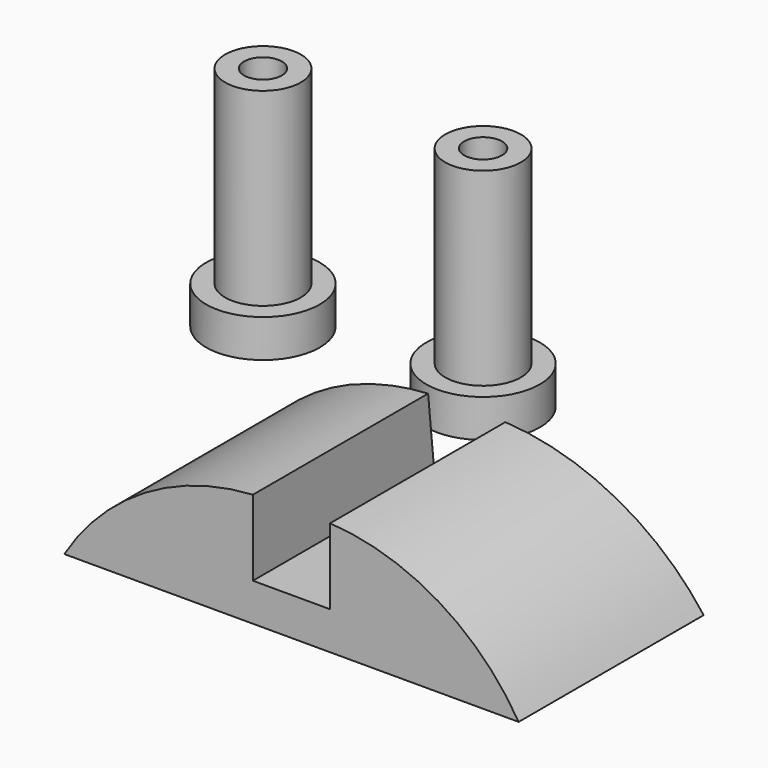
from build123d import *

# Parameters (mm, degrees)
F3_REACH = 81.3802869415
F4_R     = 6.35
F4_R_2   = 3.175
F5_DEPTH = 38.1
F6_R     = 9.525
F7_DEPTH = 6.35


with BuildPart() as f3:
    f3_end = Plane(origin=(0, 38.339396032, 4.1249082693), x_dir=(0, -0.1069719436, 0.9942620395), z_dir=(0, 0.9942620395, 0.1069719436))
    # F1 (on Front) → F3 (new body, up to a plane its end follows)
    with BuildSketch(Plane.XZ):
        with BuildLine():
            Line((0, 6.35), (0, 0))
            Line((0, 0), (38.1, 0))
            ThreePointArc((38.1, 0), (24.6352816359, 13.4206575155), (6.477, 19.05))
            Line((6.477, 19.05), (6.477, 6.35))
            Line((6.477, 6.35), (0, 6.35))
        make_face()
        with BuildLine():
            Line((-38.1, 0), (0, 0))
            Line((0, 0), (0, 6.35))
            Line((0, 6.35), (-6.477, 6.35))
            Line((-6.477, 6.35), (-6.477, 19.05))
            ThreePointArc((-6.477, 19.05), (-24.6352816359, 13.4206575155), (-38.1, 0))
        make_face()
    f3_long = extrude(amount=-F3_REACH, mode=Mode.PRIVATE)
    add(split(f3_long, bisect_by=f3_end, keep=Keep.BOTTOM, mode=Mode.PRIVATE))


with BuildPart() as f5:
    # F4 (on Top) → F5 (new body)
    with BuildSketch(Plane.XY):
        with Locations((-58.1043511629, 66.6491091251)):
            Circle(F4_R)
        with Locations((-58.1043511629, 66.6491091251)):
            Circle(F4_R_2, mode=Mode.SUBTRACT)
    extrude(amount=F5_DEPTH)


with BuildPart() as f5b:
    # F4 (on Top) → F5, piece 2 (new body)
    with BuildSketch(Plane.XY):
        with Locations((-21.4395727962, 66.9598281384)):
            Circle(F4_R)
        with Locations((-21.4395727962, 66.9598281384)):
            Circle(F4_R_2, mode=Mode.SUBTRACT)
    extrude(amount=F5_DEPTH)


with BuildPart() as f7:
    # F6 (on face) → F7 (new body)
    with BuildSketch(Plane(origin=(0, 0, 0), x_dir=(1, 0, 0), z_dir=(0, 0, -1))):
        with Locations((-58.1043511629, -66.6491091251)):
            Circle(F6_R)
    extrude(amount=-F7_DEPTH)


with BuildPart() as f7b:
    # F6 (on face) → F7, piece 2 (new body)
    with BuildSketch(Plane(origin=(0, 0, 0), x_dir=(1, 0, 0), z_dir=(0, 0, -1))):
        with Locations((-21.4395727962, -66.9598281384)):
            Circle(F6_R)
    extrude(amount=-F7_DEPTH)


solid = Compound([f3.part, f5.part, f5b.part, f7.part, f7b.part])
